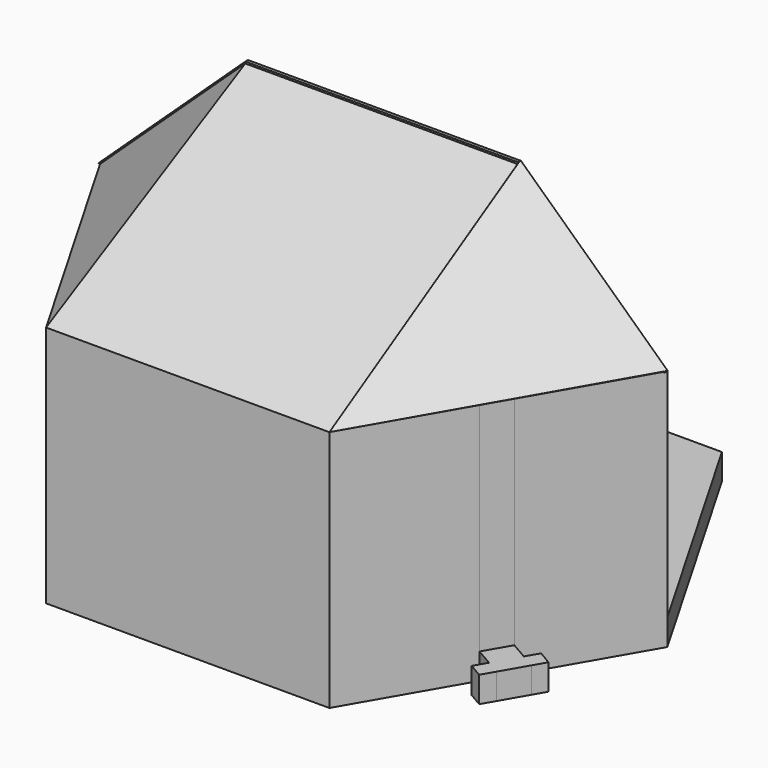
from build123d import *

# Parameters (mm, degrees)
F0_W      = 50
F0_H      = 12.5
F1_DEPTH  = 8
F2_DEPTH  = 75
F4_DEPTH  = 8
F7_DEPTH  = 3
F8_DEPTH  = 1
F11_DEPTH = 3
F14_DEPTH = 3
F15_DEPTH = 8
F16_DEPTH = 8
F17_DEPTH = 12.5
F18_DEPTH = 8


# Not quite as in the source:
# - a feature names something its author has since deleted; it is built from what else it names


with BuildPart() as f1:
    # F0 (on Top) → F1 (new body)
    with BuildSketch(Plane.XY):
        Polygon((42.0179491924, -72.7772228311), (84.0358983849, 0), (42.0179491924, 72.7772228311), (-42.0179491924, 72.7772228311), (-84.0358983849, 0), (-42.0179491924, -72.7772228311), align=None)
        with Locations((0, 54.5829171234)):
            Rectangle(F0_W, F0_H, mode=Mode.SUBTRACT)
    extrude(amount=F1_DEPTH)

    # F0 (on Top) → F2 (join)
    with BuildSketch(Plane.XY):
        Polygon((67.6939940411, -34.3050086158), (87.5, 0), (84.0358983849, 0), (42.0179491924, -72.7772228311), (-42.0179491924, -72.7772228311), (-84.0358983849, 0), (-87.5, 0), (-43.75, -75.7772228311), (43.75, -75.7772228311), (63.1939940411, -42.0992372499), align=None)
    extrude(amount=F2_DEPTH)

    # F0 (on Top) → F4 (join)
    with BuildSketch(Plane.XY):
        Polygon((43.75, 75.7772228311), (-43.75, 75.7772228311), (-65.625, 37.8886114156), (-68.125, 33.5584843966), (-87.5, 0), (-84.0358983849, 0), (-42.0179491924, 72.7772228311), (42.0179491924, 72.7772228311), (84.0358983849, 0), (87.5, 0), align=None)
    extrude(amount=F4_DEPTH)

    # F6 (on face) → F7 (join)
    with BuildSketch(Plane(origin=(0, -50.1312366318, 89.3836679776), x_dir=(1, 0, 0), z_dir=(0, 0.4891706574, -0.872188092))):
        Polygon((43.75, 29.4041920927), (0, 29.4041920927), (-43.75, 29.4041920927), (-42.01795, -57.4775522498), (42.01795, -57.4775522498), align=None)
    extrude(amount=F7_DEPTH)

    # F3 (on Front) → F8 (join)
    with BuildSketch(Plane.XZ):
        Polygon((-42.01795, 114.5), (0, 114.5), (42.01795, 114.5), (84.0359, 75), (87.5, 75), (42.01795, 117.5), (0, 117.5), (-42.01795, 117.5), (-87.5, 75), (-84.0359, 75), align=None)
    extrude(amount=F8_DEPTH)

    # F10 (on face) → F11 (join)
    with BuildSketch(Plane(origin=(-67.6846727043, -39.0777640058, 72.4338274863), x_dir=(0.7723629594, -0.3015876344, 0.5590173143), z_dir=(-0.6351814378, -0.3667221741, 0.6797495039))):
        Polygon((33.2314262259, 55.789645187), (-25.6554603702, 35.6104118215), (30.9888924807, -31.0804218073), align=None)
    extrude(amount=-F11_DEPTH)

    # F13 (on face) → F14 (join)
    with BuildSketch(Plane(origin=(67.6756688636, -39.5950852503, 72.4241918832), x_dir=(0.7733047167, 0.3041472681, -0.556322078), z_dir=(-0.6340345536, 0.3709553614, -0.6785221475))):
        Polygon((-30.939509805, 30.5117392321), (-32.8751652468, -56.3649154418), (25.9400068576, -35.9776056011), align=None)
    extrude(amount=F14_DEPTH)

    # F0 (on Top) → F15 (join)
    with BuildSketch(Plane.XY):
        with Locations((0, 54.5829171234)):
            Rectangle(F0_W, F0_H)
    extrude(amount=F15_DEPTH)

    # F0 (on Top) → F16 (join)
    with BuildSketch(Plane.XY):
        Polygon((75.395275497, -33.566783298), (73.1502941936, -37.4552049777), (77.4800811039, -39.9550086158), (79.6937291893, -36.1208576617), align=None)
        Polygon((73.1502941936, -37.4552049777), (67.6939940411, -34.3050086158), (63.1939940411, -42.0992372499), (68.6500615294, -45.249299283), (72.9800811039, -47.7492372499), (77.4800811039, -39.9550086158), align=None)
    extrude(amount=F16_DEPTH)

    # F0 (on Top) → F17 (cut, symmetric)
    with BuildSketch(Plane.XY):
        with Locations((0, 54.5829171234)):
            Rectangle(F0_W, F0_H)
    extrude(amount=F17_DEPTH, both=True, mode=Mode.SUBTRACT)

    # F0 (on Top) → F18 (join)
    with BuildSketch(Plane.XY):
        Polygon((72.9800811039, -47.7492372499), (68.6500615294, -45.249299283), (66.405071243, -49.1377365216), (70.7174794095, -51.6681783419), align=None)
    extrude(amount=F18_DEPTH)


solid = f1.part
